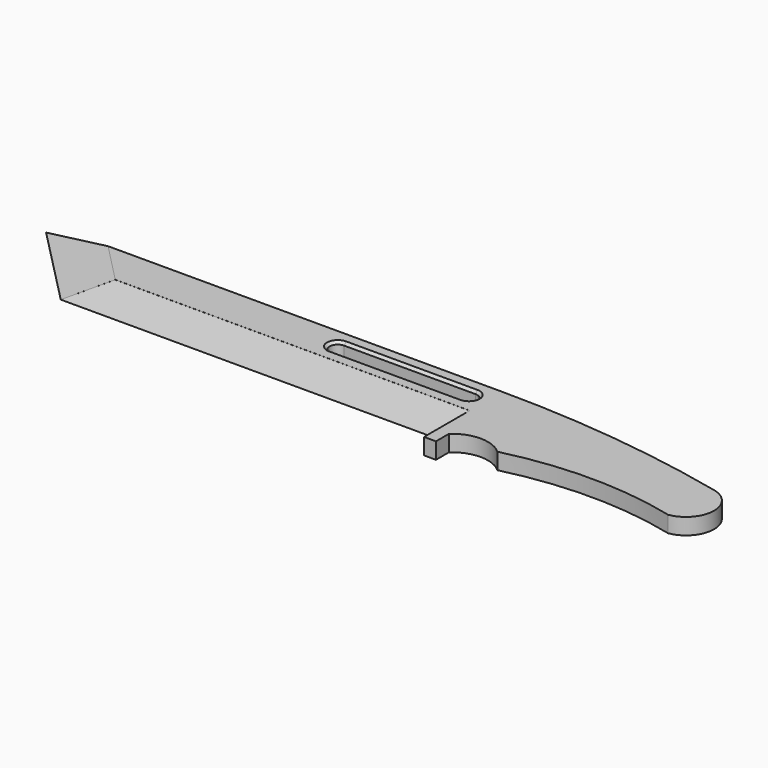
from build123d import *

# Parameters (mm, degrees)
F1_DEPTH    = 6.35
F2_DEPTH    = 6.35
F3_DEPTH    = 6.35
F4_T1_DEPTH = 229.8266509334
F5_T1_DEPTH = 134.2211036102
F6_SIZE     = 1.016


# Not quite as in the source:
# - a fillet or chamfer that OpenCascade refuses, or shapes differently, is made with other operations: its cross-section is extruded or revolved along the edge and cut away or added


with BuildPart() as f1:
    # F0 (on Top) → F1 (new body)
    with BuildSketch(Plane.XY):
        with BuildLine():
            Line((42.8011300921, 10.175053092), (-110.832311213, 10.175053092))
            Line((-110.832311213, 10.175053092), (-95.3400209546, -5.699946908))
            Line((-95.3400209546, -5.699946908), (42.8011300921, -5.699946908))
            Line((42.8011300921, -5.699946908), (42.8011300921, -21.574946908))
            Line((42.8011300921, -21.574946908), (42.8011300921, -27.924946908))
            Line((42.8011300921, -27.924946908), (47.4472232163, -27.924946908))
            Line((47.4472232163, -27.924946908), (47.4472232163, -21.574946908))
            ThreePointArc((47.4472232163, -21.574946908), (56.8993929774, -17.9668468512), (66.3515627384, -21.574946908))
            ThreePointArc((66.3515627384, -21.574946908), (99.5976924896, -17.5079847975), (132.8438222408, -21.574946908))
            ThreePointArc((132.8438222408, -21.574946908), (142.1418780211, -10.84272639), (132.9729259014, 0))
            ThreePointArc((132.9729259014, 0), (88.1731602013, 7.6232435083), (42.8011300921, 10.175053092))
        make_face()
        with BuildLine():
            Line((-14.9693377316, 5.412553092), (36.1893251538, 5.412553092))
            ThreePointArc((36.1893251538, 5.412553092), (39.3643251538, 2.237553092), (36.1893251538, -0.937446908))
            Line((36.1893251538, -0.937446908), (-14.9693377316, -0.937446908))
            ThreePointArc((-14.9693377316, -0.937446908), (-18.1443377316, 2.237553092), (-14.9693377316, 5.412553092))
        make_face(mode=Mode.SUBTRACT)
    extrude(amount=F1_DEPTH)

    # F6
    f6_edges = [f1.edges().sort_by_distance(p)[0] for p in [
        (10.609994, 5.412553, 6.35),
        (-18.144338, 2.237553, 6.35),
        (10.609994, -0.937447, 6.35),
        (39.364325, 2.237553, 6.35),
        (10.609994, -0.937447, 0),
        (-18.144338, 2.237553, 0),
        (39.364325, 2.237553, 0),
        (10.609994, 5.412553, 0),
    ]]
    chamfer(f6_edges, length=F6_SIZE)


with BuildPart() as f2:
    # F0 (on Top) → F2 (new body)
    with BuildSketch(Plane.XY):
        Polygon((-95.3400209546, -5.699946908), (-103.8739830256, -21.574946908), (42.8011300921, -21.574946908), (42.8011300921, -5.699946908), align=None)
    extrude(amount=F2_DEPTH)

    # F4: chamfer of 16.002 x 3.175 on 2 edges, made by hand

    # F4_s2 → F4_t1 (cut)
    with BuildSketch(Plane.YZ.offset(-145.4497519334)):
        Polygon((-21.574946908, 3.175), (-5.572946908, 6.35), (-21.574946908, 6.35), align=None)
        Polygon((-21.574946908, 3.175), (-5.572946908, 0), (-21.574946908, 0), align=None)
    extrude(amount=F4_T1_DEPTH, mode=Mode.SUBTRACT)


with BuildPart() as f3:
    # F0 (on Top) → F3 (new body)
    with BuildSketch(Plane.XY):
        Polygon((-110.832311213, 10.175053092), (-134.9988699079, 10.175053092), (-103.8739830256, -21.574946908), (-95.3400209546, -5.699946908), align=None)
    extrude(amount=F3_DEPTH)

    # F5: chamfer of 17.272 x 3.175 on 2 edges, made by hand

    # F5_s2 → F5_t1 (cut)
    with BuildSketch(Plane(origin=(-102.6616678748, 104.7235277465, 0), x_dir=(0, 0, 1), z_dir=(0.7000420043, -0.714101668, 0))):
        Polygon((3.175, 89.2799536123), (6.35, 72.0079536123), (6.35, 89.2799536123), align=None)
        Polygon((3.175, 89.2799536123), (0, 72.0079536123), (0, 89.2799536123), align=None)
    extrude(amount=F5_T1_DEPTH, mode=Mode.SUBTRACT)


solid = Compound([f1.part, f2.part, f3.part])
